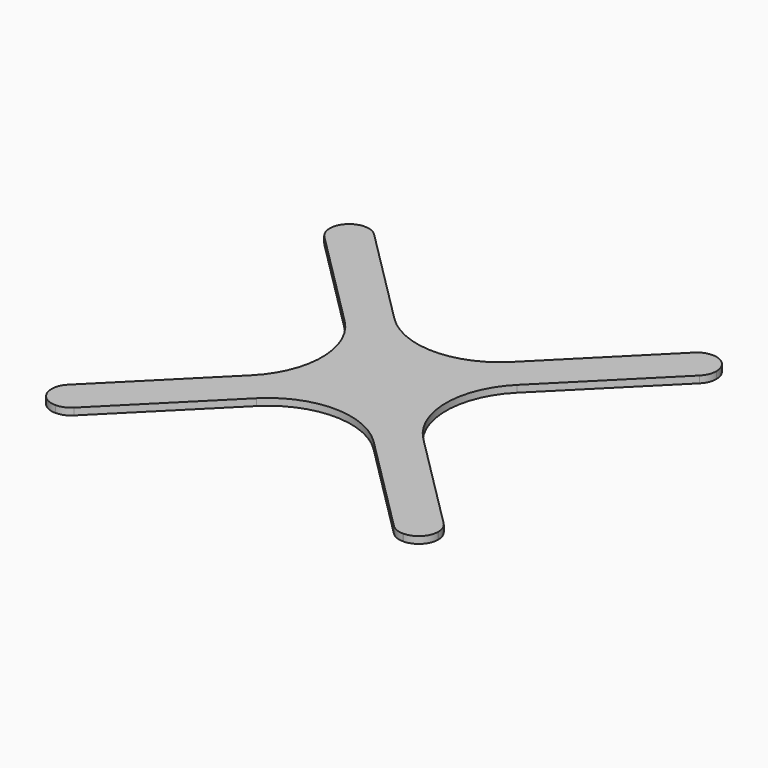
from build123d import *

# Parameters (mm, degrees)
F0_W     = 177.8
F0_H     = 177.8
F1_DEPTH = 3.175
F3_DEPTH = 3.176
F4_R     = 38.1
F5_R     = 8.89


# Not quite as in the source:
# - a length typed as a fraction of an inch, garbled in the dataset ("3 / 203.2 mm" for 3/8 in), is restored


with BuildPart() as f1:
    # F0 (on Top) → F1 (new body)
    with BuildSketch(Plane.XY):
        Rectangle(F0_W, F0_H)
    extrude(amount=F1_DEPTH)

    # F2 (on face) → F3 (cut, through all)
    with BuildSketch(Plane.XY.offset(3.175)):
        Polygon((76.2, 88.9), (-76.2, 88.9), (0, 12.7), align=None)
        Polygon((88.9, -76.2), (88.9, 76.2), (12.7, 0), align=None)
        Polygon((-76.2, -88.9), (76.2, -88.9), (0, -12.7), align=None)
        Polygon((-12.7, 0), (-88.9, 76.2), (-88.9, -76.2), align=None)
    extrude(amount=-F3_DEPTH, mode=Mode.SUBTRACT)

    # F4
    f4_edges = [f1.edges().sort_by_distance(p)[0] for p in [
        (0, -12.7, 1.5875),
        (12.7, 0, 1.5875),
        (0, 12.7, 1.5875),
        (-12.7, 0, 1.5875),
    ]]
    fillet(f4_edges, radius=F4_R)

    # F5
    f5_edges = [f1.edges().sort_by_distance(p)[0] for p in [
        (88.9, 88.9, 1.5875),
        (88.9, 76.2, 1.5875),
        (88.9, -76.2, 1.5875),
        (88.9, -88.9, 1.5875),
        (76.2, -88.9, 1.5875),
        (-76.2, -88.9, 1.5875),
        (-88.9, -88.9, 1.5875),
        (-88.9, -76.2, 1.5875),
        (-88.9, 76.2, 1.5875),
        (-88.9, 88.9, 1.5875),
        (-76.2, 88.9, 1.5875),
        (76.2, 88.9, 1.5875),
    ]]
    fillet(f5_edges, radius=F5_R)


solid = f1.part
